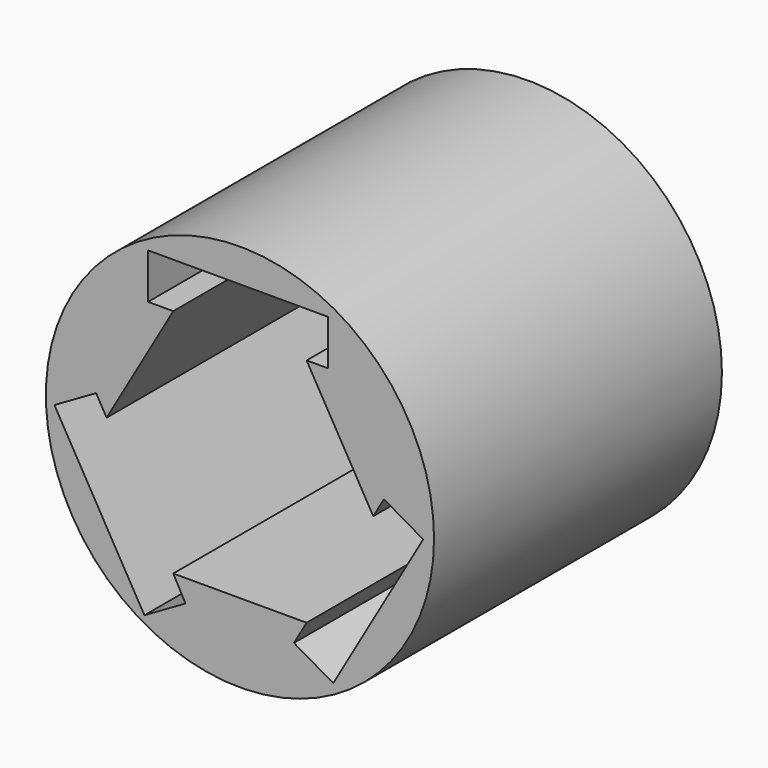
from build123d import *

# Parameters (mm, degrees)
F0_R         = 6.85
F1_DEPTH     = 12.7
F4_TEXT_SIZE = 14.5745822617
F5_DEPTH     = 1.5


# Not quite as in the source:
# - Text() gives the source's letters only with a copy of the font that has no kerning and outlines rounded to 1/6400 em; it was checked with that copy


with BuildPart() as f1:
    # F0 (on Front) → F1 (new body)
    with BuildSketch(Plane.XZ):
        Circle(F0_R)
        Polygon((2.3527023469, 4.075), (4.7054046939, 0), (5.0818449481, 0.6520136462), (6.4676587992, -0.1480863538), (3.2926587992, -5.6473476678), (1.9068449481, -4.8472476678), (2.3527023469, -4.075), (-2.3527023469, -4.075), (-1.9221597636, -4.8677240387), (-3.3717710256, -5.704657491), (-6.5467710256, -0.205396177), (-5.0768071233, 0.6432878777), (-4.7054046939, 0), (-2.3527023469, 4.075), (-3.243632324, 4.075), (-3.243632324, 5.6752), (3.106367676, 5.6752), (3.106367676, 4.075), align=None, mode=Mode.SUBTRACT)
    extrude(amount=F1_DEPTH)


with BuildPart() as f2_1:
    # F2: copy of F1
    add(f1.part)


with BuildPart() as f5_tool:
    # F4 (on offset) → F5 (new body)
    with BuildSketch(Plane.XY.offset(-7.112)):
        with Locations((-3.8882505614, -11.5696396679)):
            Text('8', F4_TEXT_SIZE, font='Open Sans', text_align=(TextAlign.LEFT, TextAlign.BOTTOM))
    extrude(amount=F5_DEPTH)


with BuildPart() as f1_1:
    add(f1.part)

    # F5: cut by f5_tool
    add(f5_tool.part, mode=Mode.SUBTRACT)


with BuildPart() as f2_1_1:
    add(f2_1.part)

    # F5: cut by f5_tool
    add(f5_tool.part, mode=Mode.SUBTRACT)


solid = Compound([f1_1.part, f2_1_1.part])
